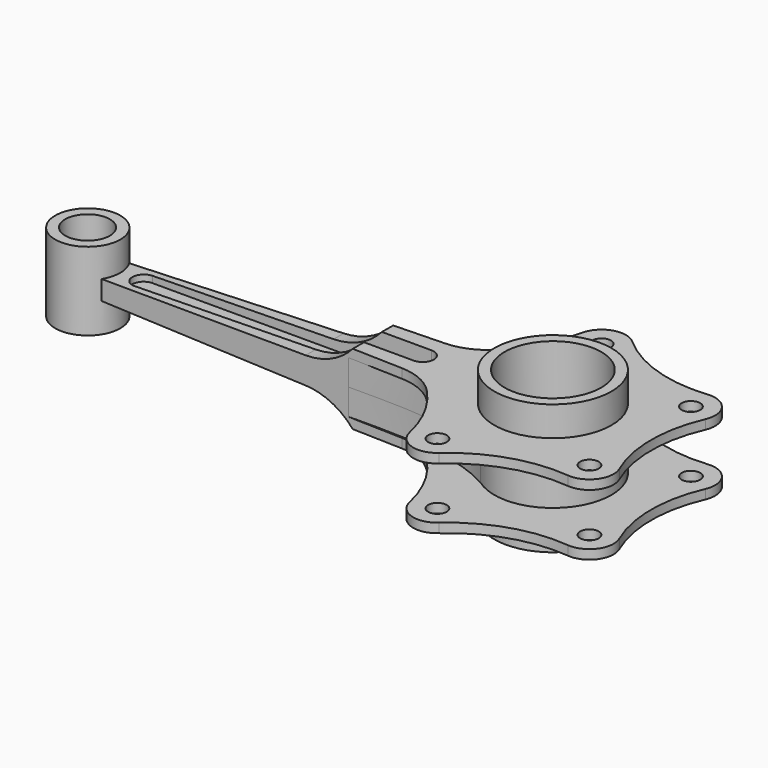
from build123d import *

# Parameters (mm, degrees)
F0_R           = 5
F1_DEPTH       = 19
F2_R           = 30
F4_DEPTH       = 68.1622779451
F4_DEPTH_BACK  = 68.1622779451
F6_DEPTH       = 17
F7_R           = 17.5
F8_DEPTH       = 21
F9_R           = 31.5
F10_DEPTH      = 35
F11_R          = 26
F11_R_2        = 12
F12_DEPTH      = 35.001
F12_DEPTH_BACK = 35.001
F14_DEPTH      = 14


# Not quite as in the source:
# - a pattern or mirror of a feature is missing from the dataset's text; its kind, count and spacing are read off the source's solid


with BuildPart() as f1:
    # F0 (on Top) → F1 (new body, symmetric)
    with BuildSketch(Plane.XY):
        with BuildLine():
            Line((-59.0811555974, 14.776369125), (-242.0627460668, 9))
            ThreePointArc((-242.0627460668, 9), (-262, 0), (-242.0627460668, -9))
            Line((-242.0627460668, -9), (-59.0811555974, -14.776369125))
            ThreePointArc((-59.0811555974, -14.776369125), (-40.8431490751, -33.7168566701), (-30.6219392979, -57.9427482129))
            ThreePointArc((-30.6219392979, -57.9427482129), (-21.9402066006, -67.525012657), (-9.2842235841, -64.8757923209))
            ThreePointArc((-9.2842235841, -64.8757923209), (16.3120043944, -50.2031873831), (45.6441286161, -47.0284888095))
            ThreePointArc((45.6441286161, -47.0284888095), (51.7840412923, -46.1484985714), (56.817332917, -42.5237384537))
            ThreePointArc((56.817332917, -42.5237384537), (57.4402066006, -41.7327529128), (58, -40.8959368627))
            ThreePointArc((58, -40.8959368627), (59.8919790803, -34.9888795877), (58.8315621696, -28.8775436891))
            ThreePointArc((58.8315621696, -28.8775436891), (52.7867550697, 0), (58.8315621696, 28.8775436891))
            ThreePointArc((58.8315621696, 28.8775436891), (57.4402066006, 41.7327529128), (45.6441286161, 47.0284888095))
            ThreePointArc((45.6441286161, 47.0284888095), (16.3120043944, 50.2031873831), (-9.2842235841, 64.8757923209))
            ThreePointArc((-9.2842235841, 64.8757923209), (-21.9402066006, 67.525012657), (-30.6219392979, 57.9427482129))
            ThreePointArc((-30.6219392979, 57.9427482129), (-40.8431490751, 33.7168566701), (-59.0811555974, 14.776369125))
        make_face()
        with Locations((-17.9229856737, -55.1612779451)):
            Circle(F0_R, mode=Mode.SUBTRACT)
        with Locations((46.9229856737, -34.091544633)):
            Circle(F0_R, mode=Mode.SUBTRACT)
        with Locations((46.9229856737, 34.091544633)):
            Circle(F0_R, mode=Mode.SUBTRACT)
        with Locations((-17.9229856737, 55.1612779451)):
            Circle(F0_R, mode=Mode.SUBTRACT)
    extrude(amount=F1_DEPTH, both=True)

    # F2
    f2_edges = [f1.edges().sort_by_distance(p)[0] for p in [
        (-59.081156, -14.776369, 0),
        (-59.081156, 14.776369, 0),
    ]]
    fillet(f2_edges, radius=F2_R)

    # F3 (on Front) → F4 (cut, two sides)
    with BuildSketch(Plane.XZ) as f4_sk:
        with BuildLine():
            Line((-263.6091709137, 30.4701216519), (-263.6091709137, 5.1802080125))
            Line((-263.6091709137, 5.1802080125), (-237.1822595596, 5.1802080125))
            Line((-237.1822595596, 5.1802080125), (-122.6608902216, 7.1397568099))
            ThreePointArc((-122.6608902216, 7.1397568099), (-107.3327979651, 10.8923192575), (-95.1225018348, 20.8893590972))
            Line((-95.1225018348, 20.8893590972), (-99.9499186873, 36.1623689532))
            Line((-99.9499186873, 36.1623689532), (-263.6091709137, 30.4701216519))
        make_face()
    f4 = extrude(amount=F4_DEPTH, mode=Mode.SUBTRACT) + extrude(f4_sk.sketch, amount=-F4_DEPTH_BACK, mode=Mode.SUBTRACT)

    # F4_copies: F4 across plane
    add(f4.mirror(Plane(origin=(0, 0, 0), x_dir=(-1, 0, 0), z_dir=(0, 0, -1))), mode=Mode.SUBTRACT)

    # F5 (on face) → F6 (cut)
    with BuildSketch(Plane.XY.offset(19)):
        with BuildLine():
            Line((-220, -6), (-96.7018583624, -6))
            Line((-96.7018583624, -6), (-96.7018583624, 6))
            Line((-96.7018583624, 6), (-220, 6))
            ThreePointArc((-220, 6), (-226, 0), (-220, -6))
        make_face()
        with BuildLine():
            Line((-96.7018583624, -6), (-70, -6))
            ThreePointArc((-70, -6), (-64, 0), (-70, 6))
            Line((-70, 6), (-96.7018583624, 6))
            Line((-96.7018583624, 6), (-96.7018583624, -6))
        make_face()
    f6 = extrude(amount=-F6_DEPTH, mode=Mode.SUBTRACT)

    # F6_copies: F6 across plane
    add(f6.mirror(Plane(origin=(0, 0, 0), x_dir=(-1, 0, 0), z_dir=(0, 0, -1))), mode=Mode.SUBTRACT)

    # F7 (on Top) → F8 (join, symmetric)
    with BuildSketch(Plane.XY):
        with Locations((-249.9698251486, 0)):
            Circle(F7_R)
    extrude(amount=F8_DEPTH, both=True)

    # F9 (on Top) → F10 (join, symmetric)
    with BuildSketch(Plane.XY):
        Circle(F9_R)
    extrude(amount=F10_DEPTH, both=True)

    # F11 (on Top) → F12 (cut, two sides)
    with BuildSketch(Plane.XY) as f12_sk:
        Circle(F11_R)
        with Locations((-250.0837445259, 0)):
            Circle(F11_R_2)
    extrude(amount=F12_DEPTH, mode=Mode.SUBTRACT)
    extrude(f12_sk.sketch, amount=-F12_DEPTH_BACK, mode=Mode.SUBTRACT)

    # F13 (on Top) → F14 (cut, symmetric)
    with BuildSketch(Plane.XY):
        with BuildLine():
            ThreePointArc((-18.3036962635, 25.6363941126), (31.5, 0), (-18.3036962635, -25.6363941126))
            add(Edge.make_bspline(
                [(-18.3036962635, -25.6363941126), (-27.5141939878, -20.3836555585), (-49.177483171, -13.7305001424), (-77.4823920391, -13.2141179704), (-99.0737920775, -13.3882725282)],
                knots=[0, 0, 0, 0, 0.437335129, 1, 1, 1, 1], degree=3))
            Line((-99.0737920775, -13.3882725282), (-70.2373236418, -76.3870328665))
            Line((-70.2373236418, -76.3870328665), (80.8955654502, -76.3870328665))
            Line((80.8955654502, -76.3870328665), (95.1919183135, 50.9186014533))
            Line((95.1919183135, 50.9186014533), (-91.0010784864, 91.0845473409))
            Line((-91.0010784864, 91.0845473409), (-99.0737920775, 13.3882725282))
            add(Edge.make_bspline(
                [(-18.3036962635, 25.6363941126), (-27.5141939878, 20.3836555585), (-49.177483171, 13.7305001424), (-77.4823920391, 13.2141179704), (-99.0737920775, 13.3882725282)],
                knots=[0, 0, 0, 0, 0.437335129, 1, 1, 1, 1], degree=3))
        make_face()
    extrude(amount=F14_DEPTH, both=True, mode=Mode.SUBTRACT)


solid = f1.part
